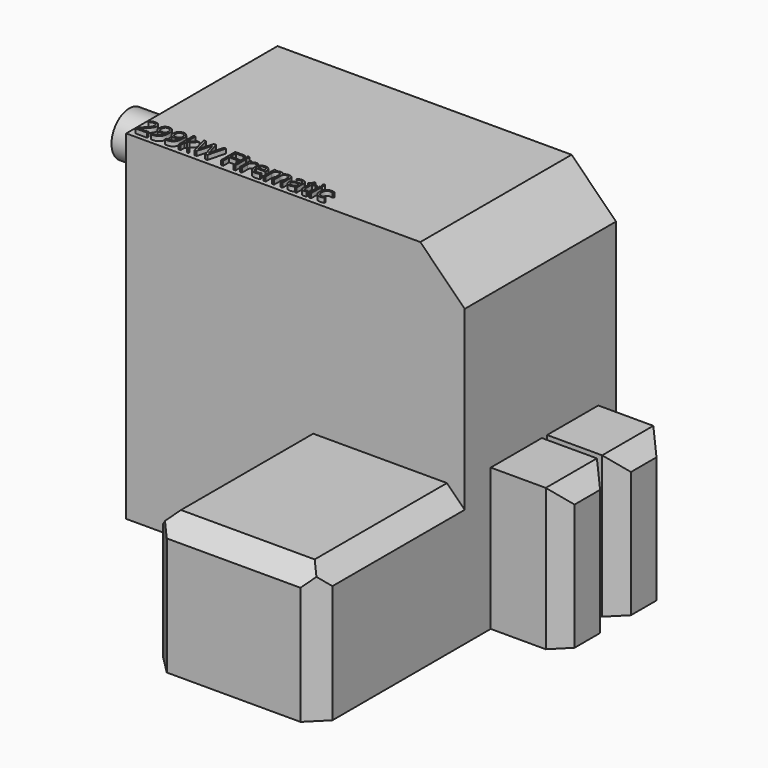
from build123d import *

# Parameters (mm, degrees)
F0_W         = 1906
F0_H         = 1065
F1_DEPTH     = 1911
F2_TEXT_SIZE = 138.8888888889
F3_DEPTH     = 25
F4_W         = 953
F4_H         = 765
F5_DEPTH     = 1031
F6_C1_SIZE   = 100
F6_C2_SIZE   = 100
F6_C3_SIZE   = 100
F6_C4_SIZE   = 100
F6_C5_SIZE   = 100
F8_W         = 360
F8_H         = 800
F9_DEPTH     = 400
F10_SIZE     = 90
F11_W        = 360
F11_H        = 800
F12_DEPTH    = 400
F13_SIZE     = 90
F14_R        = 125
F15_DEPTH    = 355
F16_SIZE     = 250


# Not quite as in the source:
# - two fillets or chamfers of one size are made in one step
# - Text() gives the source's letters only with a copy of the font that has no kerning and outlines rounded to 1/6400 em; it was checked with that copy


with BuildPart() as f1:
    # F0 (on Top) → F1 (new body)
    with BuildSketch(Plane.XY):
        with Locations((953, 532.5)):
            Rectangle(F0_W, F0_H)
    extrude(amount=F1_DEPTH)

    # F2 (on face) → F3 (join)
    with BuildSketch(Plane.XY.offset(1911)):
        with Locations((25, 25)):
            Text('299kW Firematic', F2_TEXT_SIZE, font='Open Sans', text_align=(TextAlign.LEFT, TextAlign.BOTTOM))
    extrude(amount=F3_DEPTH)

    # F4 (on face) → F5 (join)
    with BuildSketch(Plane.XZ):
        with Locations((1429.5, 382.5)):
            Rectangle(F4_W, F4_H)
    extrude(amount=F5_DEPTH)

    # F6: chamfer of 100 on 5 edges, made by hand

    # F6_c1
    f6_c1_edges = [f1.edges().sort_by_distance(p)[0] for p in [
        (1906, -1031, 382.5),
    ]]
    chamfer(f6_c1_edges, length=F6_C1_SIZE)

    # F6_c2
    f6_c2_edges = [f1.edges().sort_by_distance(p)[0] for p in [
        (1906, -465.5, 765),
    ]]
    chamfer(f6_c2_edges, length=F6_C2_SIZE)

    # F6_c3
    f6_c3_edges = [f1.edges().sort_by_distance(p)[0] for p in [
        (953, -515.5, 765),
    ]]
    chamfer(f6_c3_edges, length=F6_C3_SIZE)

    # F6_c4
    f6_c4_edges = [f1.edges().sort_by_distance(p)[0] for p in [
        (1429.5, -1031, 765),
    ]]
    chamfer(f6_c4_edges, length=F6_C4_SIZE)

    # F6_c5
    f6_c5_edges = [f1.edges().sort_by_distance(p)[0] for p in [
        (953, -1031, 332.5),
    ]]
    chamfer(f6_c5_edges, length=F6_C5_SIZE)

    # F8 (on face) → F9 (join)
    with BuildSketch(Plane.YZ.offset(1906)):
        with Locations((363, 400)):
            Rectangle(F8_W, F8_H)
    extrude(amount=F9_DEPTH)

    # F10
    f10_edges = [f1.edges().sort_by_distance(p)[0] for p in [
        (2306, 183, 400),
        (2306, 363, 800),
        (2306, 543, 400),
    ]]
    chamfer(f10_edges, length=F10_SIZE)

    # F11 (on face) → F12 (join, through all)
    with BuildSketch(Plane.YZ.offset(1906)):
        with Locations((760, 400)):
            Rectangle(F11_W, F11_H)
    extrude(amount=F12_DEPTH)

    # F13
    f13_edges = [f1.edges().sort_by_distance(p)[0] for p in [
        (2306, 940, 400),
        (2306, 760, 800),
        (2306, 580, 400),
    ]]
    chamfer(f13_edges, length=F13_SIZE)

    # F14 (on face) → F15 (join)
    with BuildSketch(Plane(origin=(0, 0, 0), x_dir=(0, -1, 0), z_dir=(-1, 0, 0))):
        with Locations((-465, 1606)):
            Circle(F14_R)
    extrude(amount=F15_DEPTH)

    # F16
    f16_edges = [f1.edges().sort_by_distance(p)[0] for p in [
        (1906, 532.5, 1911),
    ]]
    chamfer(f16_edges, length=F16_SIZE)


solid = f1.part
